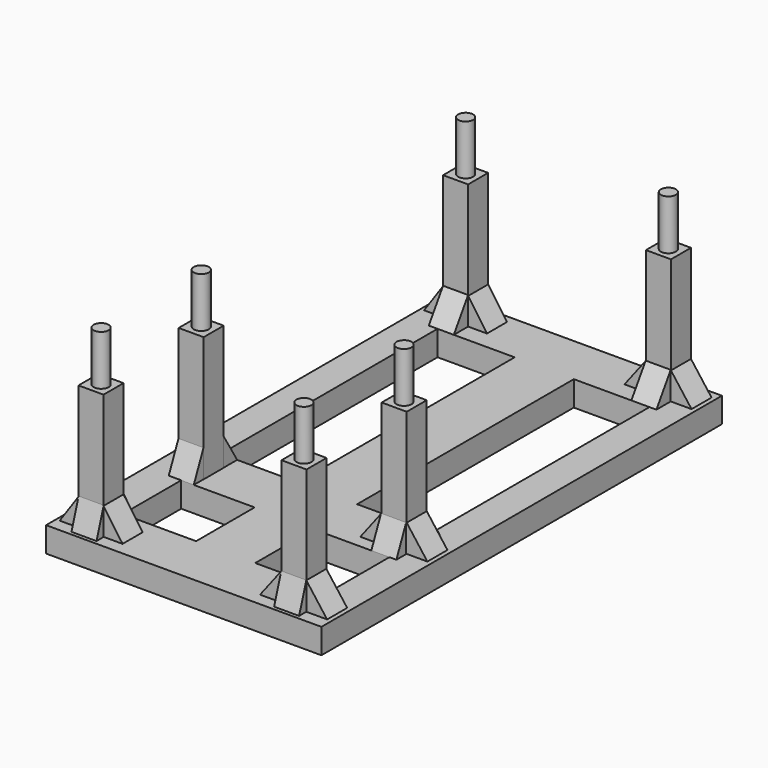
from build123d import *

# Parameters (mm, degrees)
F0_W      = 6.2445142865
F0_H      = 54.1005749255
F0_W_2    = 5
F0_H_2    = 5
F0_W_3    = 11.8177030236
F0_H_3    = 10.0689709187
F0_W_4    = 6.4211731404
F0_H_4    = 10.8302235603
F0_H_5    = 14.6082099527
F0_H_6    = 10.3920206428
F0_W_5    = 6.9924706221
F1_DEPTH  = 5
F0_R      = 1.5
F2_DEPTH  = 30
F3_DEPTH  = 40
F5_DEPTH  = 5
F7_DEPTH  = 5
F9_DEPTH  = 5
F11_DEPTH = 5
F13_DEPTH = 5


# Not quite as in the source:
# - a feature names something its author has since deleted; it is built from what else it names


with BuildPart() as f1:
    # F0 (on Top) → F1 (new body)
    with BuildSketch(Plane.XY):
        with Locations((-24.3777428567, 12.8807416186)):
            Rectangle(F0_W, F0_H)
        Polygon((-21.2554857135, 39.9310290813), (-5.8475900441, 39.9310290813), (-5.8475900441, 50), (-27.5, 50), (-27.5, 39.9310290813), align=None)
        with Locations((-20.5, 46)):
            Rectangle(F0_W_2, F0_H_2, mode=Mode.SUBTRACT)
        with Locations((0.0612614676, 44.9655145407)):
            Rectangle(F0_W_3, F0_H_3)
        Polygon((21.0788268596, 39.9310290813), (27.5, 39.9310290813), (27.5, 50), (5.9701129794, 50), (5.9701129794, 39.9310290813), align=None)
        with Locations((20.0169440359, 46.0017099977)):
            Rectangle(F0_W_2, F0_H_2, mode=Mode.SUBTRACT)
        with Locations((24.2894134298, 12.8807416186)):
            Rectangle(F0_W_4, F0_H)
        with Locations((0.0612614676, 12.8807416186)):
            Rectangle(F0_W_3, F0_H)
        with Locations((0.0612614676, -19.5846576244)):
            Rectangle(F0_W_3, F0_H_4)
        with Locations((0.0612614676, -32.3038743809)):
            Rectangle(F0_W_3, F0_H_5)
        with Locations((0.0612614676, -44.8039896786)):
            Rectangle(F0_W_3, F0_H_6)
        Polygon((5.9701129794, -50), (27.5, -50), (27.5, -39.6079793572), (21.0788268596, -39.6079793572), (5.9701129794, -39.6079793572), align=None)
        with Locations((19.9717525393, -44.9374727905)):
            Rectangle(F0_W_2, F0_H_2, mode=Mode.SUBTRACT)
        Polygon((-27.5, -50), (-5.8475900441, -50), (-5.8475900441, -39.6079793572), (-20.5075293779, -39.6079793572), (-27.5, -39.6079793572), align=None)
        with Locations((-20.5385480076, -44.9859946966)):
            Rectangle(F0_W_2, F0_H_2, mode=Mode.SUBTRACT)
        with Locations((-24.003764689, -32.3038743809)):
            Rectangle(F0_W_5, F0_H_5)
        with Locations((24.2894134298, -32.3038743809)):
            Rectangle(F0_W_4, F0_H_5)
        Polygon((21.0788268596, -24.9997694045), (27.5, -24.9997694045), (27.5, -14.1695458442), (21.0788268596, -14.1695458442), (5.9701129794, -14.1695458442), (5.9701129794, -24.9997694045), align=None)
        with Locations((19.9943464249, -19.9489668012)):
            Rectangle(F0_W_2, F0_H_2, mode=Mode.SUBTRACT)
        Polygon((-20.5075293779, -24.9997694045), (-5.8475900441, -24.9997694045), (-5.8475900441, -14.1695458442), (-21.2554857135, -14.1695458442), (-27.5, -14.1695458442), (-27.5, -24.9997694045), align=None)
        with Locations((-20.4707719386, -20.0652703643)):
            Rectangle(F0_W_2, F0_H_2, mode=Mode.SUBTRACT)
    extrude(amount=F1_DEPTH)

    # F0 (on Top) → F2 (join)
    with BuildSketch(Plane.XY):
        with Locations((-20.5, 46)):
            Rectangle(F0_W_2, F0_H_2)
        with Locations((-20.5, 46)):
            Circle(F0_R, mode=Mode.SUBTRACT)
        with Locations((20.0169440359, 46.0017099977)):
            Rectangle(F0_W_2, F0_H_2)
        with Locations((20, 46)):
            Circle(F0_R, mode=Mode.SUBTRACT)
        with Locations((-20.4707719386, -20.0652703643)):
            Rectangle(F0_W_2, F0_H_2)
        with Locations((-20.5, -20)):
            Circle(F0_R, mode=Mode.SUBTRACT)
        with Locations((19.9943464249, -19.9489668012)):
            Rectangle(F0_W_2, F0_H_2)
        with Locations((20, -20)):
            Circle(F0_R, mode=Mode.SUBTRACT)
        with Locations((19.9717525393, -44.9374727905)):
            Rectangle(F0_W_2, F0_H_2)
        with Locations((20, -45)):
            Circle(F0_R, mode=Mode.SUBTRACT)
        with Locations((-20.5385480076, -44.9859946966)):
            Rectangle(F0_W_2, F0_H_2)
        with Locations((-20.5, -45)):
            Circle(F0_R, mode=Mode.SUBTRACT)
    extrude(amount=F2_DEPTH)

    # F0 (on Top) → F3 (join)
    with BuildSketch(Plane.XY):
        with Locations((-20.5, 46)):
            Circle(F0_R)
        with Locations((20, 46)):
            Circle(F0_R)
        with Locations((20, -20)):
            Circle(F0_R)
        with Locations((-20.5, -20)):
            Circle(F0_R)
        with Locations((-20.5, -45)):
            Circle(F0_R)
        with Locations((20, -45)):
            Circle(F0_R)
    extrude(amount=F3_DEPTH)


with BuildPart() as f5:
    # F4 (on face) → F5 (new body)
    with BuildSketch(Plane.XZ.offset(47.4859946966)):
        Polygon((-23.0385480076, 5), (-23.0385480076, 10.4398299009), (-27.1731745452, 4.4442578219), (-23.0385480076, 4.4442578219), (-18.0385480076, 4.4442578219), (-13.8439134623, 4.4442578219), (-18.0385480076, 10.4398299009), (-18.0385480076, 5), align=None)
    extrude(amount=-F5_DEPTH)


with BuildPart() as f5b:
    # F4 (on face) → F5, piece 2 (new body)
    with BuildSketch(Plane.XZ.offset(47.4859946966)):
        Polygon((12.8417154774, 4.4902400114), (17.4717525393, 4.4902400114), (17.4717525393, 10.5195268989), align=None)
    extrude(amount=-F5_DEPTH)


with BuildPart() as f5c:
    # F4 (on face) → F5, piece 3 (new body)
    with BuildSketch(Plane.XZ.offset(47.4859946966)):
        Polygon((22.4717525393, 10.5195268989), (22.4717525393, 4.4902400114), (27.0158294588, 4.4902400114), align=None)
    extrude(amount=-F5_DEPTH)


with BuildPart() as f7:
    # F6 (on face) → F7 (new body)
    with BuildSketch(Plane(origin=(-23, 0, 0), x_dir=(0, -1, 0), z_dir=(-1, 0, 0))):
        Polygon((49.2872789123, 5), (47.4859946966, 10.5548109859), (47.4859946966, 5), align=None)
    extrude(amount=-F7_DEPTH)


with BuildPart() as f7b:
    # F6 (on face) → F7, piece 2 (new body)
    with BuildSketch(Plane(origin=(-23, 0, 0), x_dir=(0, -1, 0), z_dir=(-1, 0, 0))):
        Polygon((42.4859946966, 5), (42.4859946966, 10.5548109859), (39.6079793572, 5), align=None)
    extrude(amount=-F7_DEPTH)


with BuildPart() as f7c:
    # F6 (on face) → F7, piece 3 (new body)
    with BuildSketch(Plane(origin=(-23, 0, 0), x_dir=(0, -1, 0), z_dir=(-1, 0, 0))):
        Polygon((22.5652703643, 10.5548109859), (22.5652703643, 5), (24.9997694045, 5), align=None)
    extrude(amount=-F7_DEPTH)


with BuildPart() as f7d:
    # F6 (on face) → F7, piece 4 (new body)
    with BuildSketch(Plane(origin=(-23, 0, 0), x_dir=(0, -1, 0), z_dir=(-1, 0, 0))):
        Polygon((14.1695458442, 5), (17.5652703643, 5), (17.5652703643, 10.5548109859), align=None)
    extrude(amount=-F7_DEPTH)


with BuildPart() as f7e:
    # F6 (on face) → F7, piece 5 (new body)
    with BuildSketch(Plane(origin=(-23, 0, 0), x_dir=(0, -1, 0), z_dir=(-1, 0, 0))):
        Polygon((-39.9310290813, 5), (-43.5, 10.5548109859), (-43.5, 5), align=None)
    extrude(amount=-F7_DEPTH)


with BuildPart() as f7f:
    # F6 (on face) → F7, piece 6 (new body)
    with BuildSketch(Plane(origin=(-23, 0, 0), x_dir=(0, -1, 0), z_dir=(-1, 0, 0))):
        Polygon((-48.5, 5), (-48.5, 10.5548109859), (-49.4102165648, 5), align=None)
    extrude(amount=-F7_DEPTH)


with BuildPart() as f9:
    # F8 (on face) → F9 (new body)
    with BuildSketch(Plane.YZ.offset(22.4717525393)):
        Polygon((-49.2872789123, 5), (-47.4859946966, 5), (-47.4859946966, 10.5548109859), align=None)
    extrude(amount=-F9_DEPTH)


with BuildPart() as f9b:
    # F8 (on face) → F9, piece 2 (new body)
    with BuildSketch(Plane.YZ.offset(22.4717525393)):
        Polygon((-39.6079793572, 5), (-42.4374727905, 10.4611596375), (-42.4374727905, 5), align=None)
    extrude(amount=-F9_DEPTH)


with BuildPart() as f9c:
    # F8 (on face) → F9, piece 3 (new body)
    with BuildSketch(Plane.YZ.offset(22.4717525393)):
        Polygon((-22.5652703643, 10.5548109859), (-24.9997694045, 5), (-22.5652703643, 5), align=None)
    extrude(amount=-F9_DEPTH)


with BuildPart() as f9d:
    # F8 (on face) → F9, piece 4 (new body)
    with BuildSketch(Plane.YZ.offset(22.4717525393)):
        Polygon((-14.1695458442, 5), (-17.5652703643, 10.5548109859), (-17.5652703643, 5), align=None)
    extrude(amount=-F9_DEPTH)


with BuildPart() as f9e:
    # F8 (on face) → F9, piece 5 (new body)
    with BuildSketch(Plane.YZ.offset(22.4717525393)):
        Polygon((43.5, 10.5548109859), (39.9310290813, 5), (43.5, 5), align=None)
    extrude(amount=-F9_DEPTH)


with BuildPart() as f9f:
    # F8 (on face) → F9, piece 6 (new body)
    with BuildSketch(Plane.YZ.offset(22.4717525393)):
        Polygon((48.5, 5), (49.4102165648, 5), (48.5, 10.5548109859), align=None)
    extrude(amount=-F9_DEPTH)


with BuildPart() as f11:
    # F10 (on face) → F11 (new body)
    with BuildSketch(Plane(origin=(0, -17.4489668012, 0), x_dir=(-1, 0, 0), z_dir=(0, 1, 0))):
        Polygon((-22.4943464249, 5), (-22.4943464249, 10.4895483089), (-27.0158294588, 4.4902400114), (-22.4717525393, 4.4902400114), (-22.4717525393, 5), align=None)
    extrude(amount=-F11_DEPTH)


with BuildPart() as f11b:
    # F10 (on face) → F11, piece 2 (new body)
    with BuildSketch(Plane(origin=(0, -17.4489668012, 0), x_dir=(-1, 0, 0), z_dir=(0, 1, 0))):
        Polygon((-17.4717525393, 4.4902400114), (-12.8417154774, 4.4902400114), (-17.4717525393, 10.5195268989), align=None)
    extrude(amount=-F11_DEPTH)


with BuildPart() as f13:
    # F12 (on face) → F13 (new body)
    with BuildSketch(Plane(origin=(0, 48.5017099977, 0), x_dir=(-1, 0, 0), z_dir=(0, 1, 0))):
        Polygon((-22.5169440359, 5), (-22.5169440359, 10.4595647761), (-27.0158294588, 4.4902400114), (-22.4943464249, 4.4902400114), (-22.4943464249, 5), align=None)
    extrude(amount=-F13_DEPTH)


with BuildPart() as f13b:
    # F12 (on face) → F13, piece 2 (new body)
    with BuildSketch(Plane(origin=(0, 48.5017099977, 0), x_dir=(-1, 0, 0), z_dir=(0, 1, 0))):
        Polygon((-12.8417154774, 4.4902400114), (-17.4717525393, 10.5195268989), (-17.4717525393, 4.4902400114), align=None)
    extrude(amount=-F13_DEPTH)


with BuildPart() as f13c:
    # F12 (on face) → F13, piece 3 (new body)
    with BuildSketch(Plane(origin=(0, 48.5017099977, 0), x_dir=(-1, 0, 0), z_dir=(0, 1, 0))):
        Polygon((13.8439134623, 4.4442578219), (18.0385480076, 4.4442578219), (18.0385480076, 10.4398299009), align=None)
    extrude(amount=-F13_DEPTH)


with BuildPart() as f13d:
    # F12 (on face) → F13, piece 4 (new body)
    with BuildSketch(Plane(origin=(0, 48.5017099977, 0), x_dir=(-1, 0, 0), z_dir=(0, 1, 0))):
        Polygon((27.1731745452, 4.4442578219), (23.0385480076, 10.4398299009), (23.0385480076, 4.4442578219), align=None)
    extrude(amount=-F13_DEPTH)


solid = Compound([f1.part, f5.part, f5b.part, f5c.part, f7.part, f7b.part, f7c.part, f7d.part, f7e.part, f7f.part, f9.part, f9b.part, f9c.part, f9d.part, f9e.part, f9f.part, f11.part, f11b.part, f13.part, f13b.part, f13c.part, f13d.part])
